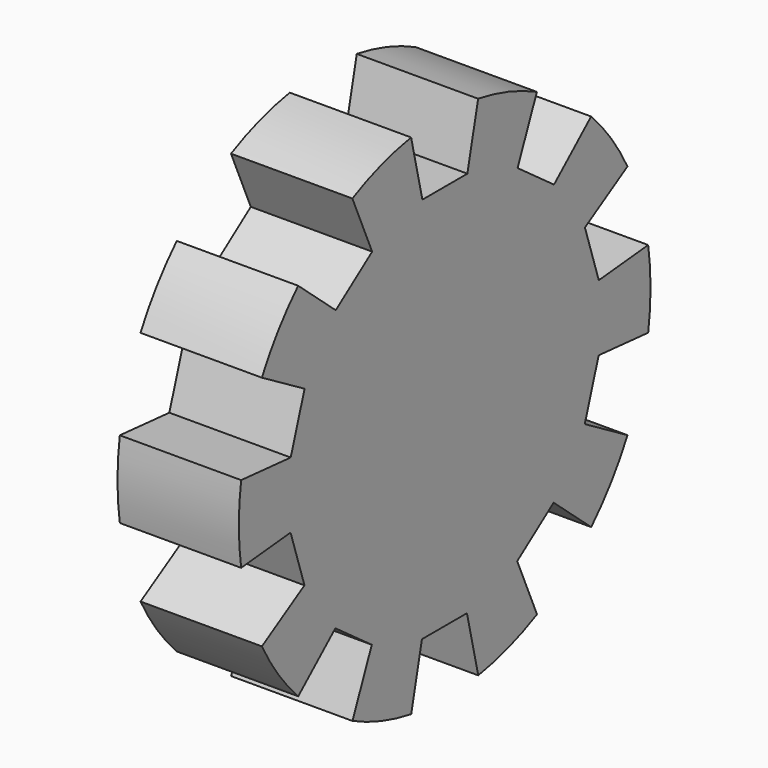
from build123d import *

# Parameters (mm, degrees)
F0_W            = 17.96984524
F0_H            = 38.1
F3_DEPTH        = 25.4
F3_COPIES_COUNT = 10


# Not quite as in the source:
# - a pattern or mirror of a feature is missing from the dataset's text; its kind, count and spacing are read off the source's solid


with BuildPart() as f1:
    # F0 (on Front) → F1 (revolve)
    with BuildSketch(Plane.XZ):
        with Locations((-8.98492262, 22.0940720202)):
            Rectangle(F0_W, F0_H)
    revolve(axis=Axis((-8.98492262, 0, 3.0440720202), (1, 0, 0)))

    # F2 (on face) → F3 (cut)
    with BuildSketch(Plane.YZ):
        with BuildLine():
            Line((-6.214665944, 40.6338036926), (-4.1235210374, 31.6734537482))
            Line((-4.1235210374, 31.6734537482), (0, 31.6734537482))
            Line((0, 31.6734537482), (0, 41.1440720202))
            ThreePointArc((0, 41.1440720202), (-3.117789544, 41.0162906591), (-6.214665944, 40.6338036926))
        make_face()
        with BuildLine():
            Line((0, 41.1440720202), (0, 31.6734537482))
            Line((0, 31.6734537482), (4.2036371306, 31.6734537482))
            Line((4.2036371306, 31.6734537482), (6.1898369976, 40.6379002098))
            ThreePointArc((6.1898369976, 40.6379002098), (3.1052492637, 41.0173182208), (0, 41.1440720202))
        make_face()
    f3 = extrude(amount=-F3_DEPTH, mode=Mode.SUBTRACT)

    # F3_copies: F3 ×10 about axis
    f3_copies_axis = Axis((0, 0, 3.044072), (1, 0, 0))
    for i in range(1, F3_COPIES_COUNT):
        add(f3.rotate(f3_copies_axis, i * 360 / F3_COPIES_COUNT), mode=Mode.SUBTRACT)


solid = f1.part
